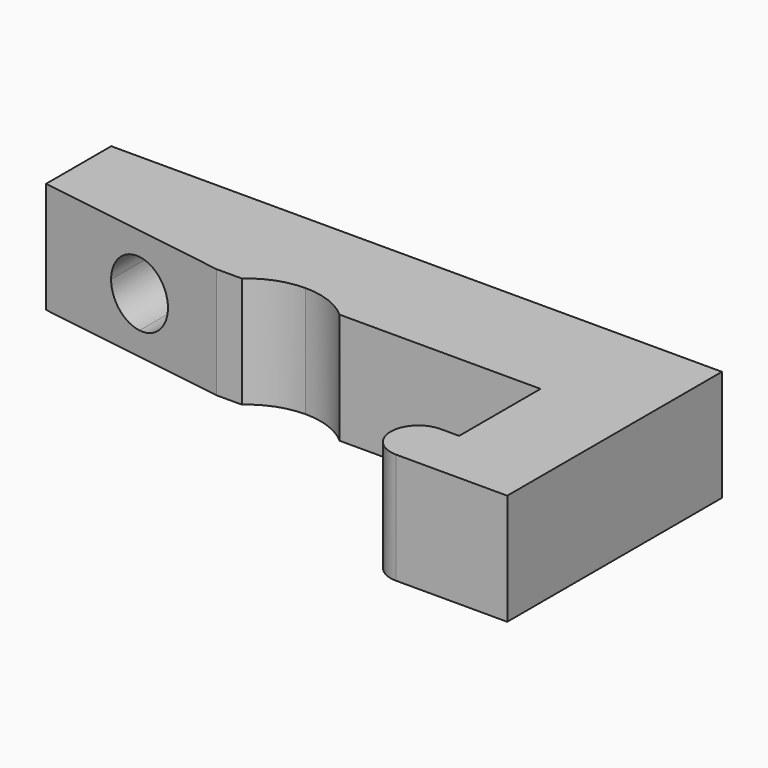
from build123d import *

# Parameters (mm, degrees)
F1_DEPTH    = 6
F3_DEPTH    = 25
F4_T1_DEPTH = 60.5769524325


# Not quite as in the source:
# - a fillet or chamfer that OpenCascade refuses, or shapes differently, is made with other operations: its cross-section is extruded or revolved along the edge and cut away or added
# - a feature names something its author has since deleted; it is built from what else it names


with BuildPart() as f1:
    # F0 (on Top) → F1 (new body)
    with BuildSketch(Plane.XY):
        with BuildLine():
            Line((-1, 0), (0, 0))
            Line((0, 0), (5, 0))
            Line((5, 0), (5, 14.5))
            Line((5, 14.5), (-28, 14.5))
            Line((-28, 14.5), (-28, 9.5))
            Line((-28, 9.5), (-13.5, 9.5))
            Line((-13.5, 9.5), (0, 9.5))
            Line((0, 9.5), (0, 8.5))
            Line((0, 8.5), (0, 3))
            Line((0, 3), (-1, 3))
            ThreePointArc((-1, 3), (-2.5, 1.5), (-1, 0))
        make_face()
        with BuildLine():
            Line((-10.8542486889, 8.5), (0, 8.5))
            Line((0, 8.5), (0, 9.5))
            Line((0, 9.5), (-13.5, 9.5))
            ThreePointArc((-13.5, 9.5), (-12.0857864376, 9.2416573868), (-10.8542486889, 8.5))
        make_face()
        with BuildLine():
            Line((-13.5, 9.5), (-28, 9.5))
            Line((-28, 9.5), (-28, 8.5))
            Line((-28, 8.5), (-16.1457513111, 8.5))
            ThreePointArc((-16.1457513111, 8.5), (-14.9142135624, 9.2416573868), (-13.5, 9.5))
        make_face()
    extrude(amount=F1_DEPTH)

    # F2 (on face) → F3 (cut)
    with BuildSketch(Plane(origin=(0, 14.5, 0), x_dir=(-1, 0, 0), z_dir=(0, 1, 0))):
        with BuildLine():
            ThreePointArc((22.25, 1.25), (23.4874368671, 1.7625631329), (24, 3))
            ThreePointArc((24, 3), (23.4874368671, 4.2374368671), (22.25, 4.75))
            Line((22.25, 4.75), (22.25, 1.25))
        make_face()
        with BuildLine():
            Line((22.25, 1.25), (22.25, 4.75))
            ThreePointArc((22.25, 4.75), (20.5, 3), (22.25, 1.25))
        make_face()
    extrude(amount=-F3_DEPTH, mode=Mode.SUBTRACT)

    # F4: chamfer of 10.5 x 1.6 on 1 edges, made by hand

    # F4_s2 → F4_t1 (cut)
    with BuildSketch(Plane.XY.offset(-27.2884762162)):
        Polygon((-28, 10.1), (-17.5, 8.5), (-28, 8.5), align=None)
    extrude(amount=F4_T1_DEPTH, mode=Mode.SUBTRACT)


solid = f1.part
